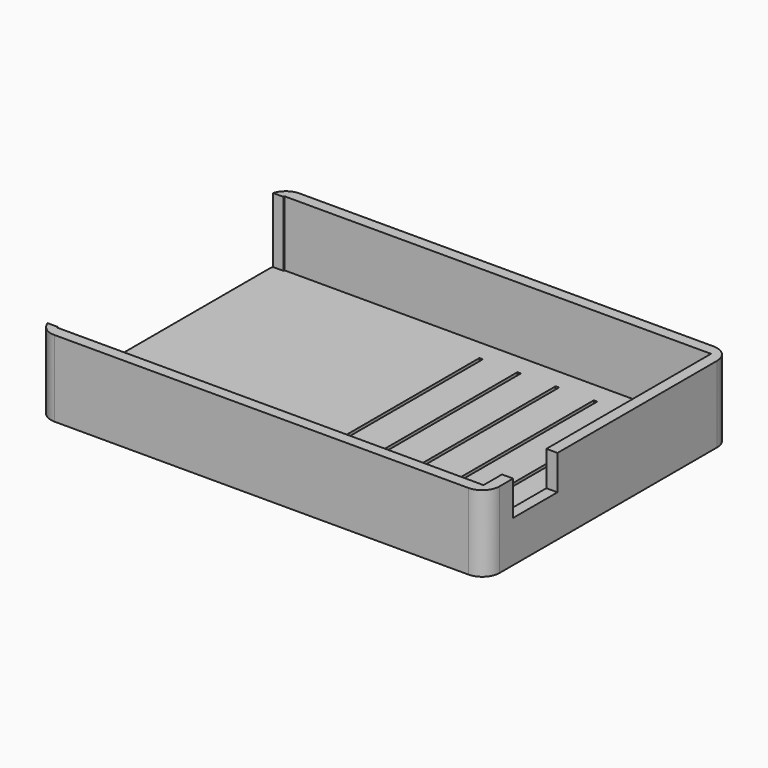
from build123d import *

# Parameters (mm, degrees)
F0_W      = 60.5
F0_H      = 40.64
F1_DEPTH  = 12.7
F2_W      = 64.6999999881
F2_H      = 44.1999999881
F2_W_2    = 61.5
F2_H_2    = 41
F3_DEPTH  = 11
F4_DEPTH  = 1.6
F5_DEPTH  = 8.8
F6_W      = 0.5
F6_H      = 35
F7_DEPTH  = 16
F8_DEPTH  = 60.7
F9_R      = 2.5
F10_R     = 2.5
F11_W     = 8
F11_H     = 5
F12_DEPTH = 1.71


# Not quite as in the source:
# - a feature names something its author has since deleted; it is built from what else it names


with BuildPart() as f1:
    # F0 (on Top) → F1 (new body)
    with BuildSketch(Plane.XY):
        Rectangle(F0_W, F0_H)
    extrude(amount=F1_DEPTH)



with BuildPart() as f3:
    # F2 (on Top) → F3 (new body)
    with BuildSketch(Plane.XY):
        Rectangle(F2_W, F2_H)
        Rectangle(F2_W_2, F2_H_2, mode=Mode.SUBTRACT)
    extrude(amount=F3_DEPTH)


with BuildPart() as f1_1:
    add(f1.part)

    add(f3.part)  # F4 merges F3
    # F2 (on Top) → F4 (join)
    with BuildSketch(Plane.XY):
        Rectangle(F2_W_2, F2_H_2)
    extrude(amount=F4_DEPTH)

    # F5 (cut): a face of the model
    f5_faces = [f1_1.faces().sort_by_distance(p)[0] for p in [
        (-30.25, 0, 7.15),
    ]]
    extrude(f5_faces, amount=F5_DEPTH, mode=Mode.SUBTRACT)

    # F6 (on face) → F7 (cut)
    with BuildSketch(Plane(origin=(0, 0, 0), x_dir=(1, 0, 0), z_dir=(0, 0, -1))):
        with Locations((22, 0)):
            Rectangle(F6_W, F6_H)
        with Locations((16.5, 0)):
            Rectangle(F6_W, F6_H)
        with Locations((11, 0)):
            Rectangle(F6_W, F6_H)
        with Locations((5.5, 0)):
            Rectangle(F6_W, F6_H)
        Rectangle(F6_W, F6_H)
    extrude(amount=-F7_DEPTH, mode=Mode.SUBTRACT)

    # F8 (cut): a face of the model
    f8_faces = [f1_1.faces().sort_by_distance(p)[0] for p in [
        (-30.25, 0, 7.15),
    ]]
    extrude(f8_faces, amount=-F8_DEPTH, mode=Mode.SUBTRACT)

    # F9
    f9_edges = [f1_1.edges().sort_by_distance(p)[0] for p in [
        (32.35, 22.1, 5.5),
        (32.35, -22.1, 5.5),
    ]]
    fillet(f9_edges, radius=F9_R)

    # F10
    f10_edges = [f1_1.edges().sort_by_distance(p)[0] for p in [
        (-32.35, 22.1, 5.5),
        (-32.35, -22.1, 5.5),
    ]]
    fillet(f10_edges, radius=F10_R)

    # F14: F12 across plane


with BuildPart() as f12:
    # F11 (on face) → F12 (new body)
    with BuildSketch(Plane.YZ.offset(32.349999994)):
        with Locations((13.1696772724, 8.5)):
            Rectangle(F11_W, F11_H)
    extrude(amount=-F12_DEPTH)


with BuildPart() as f1_2:
    add(f1_1.part)
    add(f12.part.mirror(Plane(origin=(0, 0, 5.5), x_dir=(-1, 0, 0), z_dir=(0, 1, 0))), mode=Mode.SUBTRACT)


solid = f1_2.part
